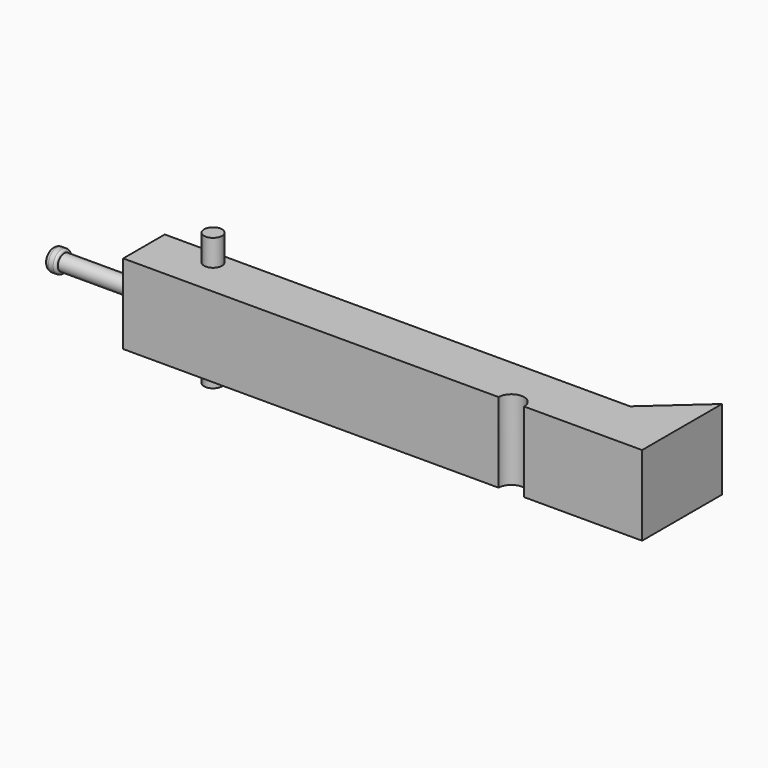
from build123d import *

# Parameters (mm, degrees)
F0_W          = 165.1
F0_H          = 25.4
F1_DEPTH      = 16.51
F3_R          = 2.8575
F4_DEPTH      = 8.382
F4_DEPTH_BACK = 33.782
F5_DEPTH      = 25.4
F6_DEPTH      = 25.4
F7_R          = 4.064
F8_DEPTH      = 25.4
F9_R          = 2.54
F10_DEPTH     = 25.4
F11_R         = 3.429
F12_DEPTH     = 3.81
F13_R         = 1.524
F14_R         = 0.762


# Not quite as in the source:
# - a feature names something its author has since deleted; it is built from what else it names


with BuildPart() as f1:
    # F0 (on Front) → F1 (new body)
    with BuildSketch(Plane.XZ):
        with Locations((17.2861106694, 1.5442719363)):
            Rectangle(F0_W, F0_H)
    extrude(amount=F1_DEPTH)

    # F3 (on face) → F4 (join, two sides)
    with BuildSketch(Plane(origin=(0, 0, -11.1557280637), x_dir=(1, 0, 0), z_dir=(0, 0, -1))) as f4_sk:
        with Locations((-46.4608334005, 4.2803706601)):
            Circle(F3_R)
    extrude(amount=F4_DEPTH)
    extrude(f4_sk.sketch, amount=-F4_DEPTH_BACK)

    # F2 (on face) → F5 (join)
    with BuildSketch(Plane(origin=(0, 0, -11.1557280637), x_dir=(1, 0, 0), z_dir=(0, 0, -1))):
        Polygon((99.8361106694, 0), (82.7972726808, 0), (99.8361106694, -15.24), align=None)
    extrude(amount=-F5_DEPTH)

    # F2 (on face) → F6 (join)
    with BuildSketch(Plane(origin=(0, 0, -11.1557280637), x_dir=(1, 0, 0), z_dir=(0, 0, -1))):
        Polygon((99.8361106694, 0), (82.7972726808, 0), (99.8361106694, -15.24), align=None)
    extrude(amount=-F6_DEPTH)

    # F7 (on face) → F8 (cut)
    with BuildSketch(Plane(origin=(0, 0, -11.1557280637), x_dir=(1, 0, 0), z_dir=(0, 0, -1))):
        with Locations((58.2425315266, 16.51)):
            Circle(F7_R)
    extrude(amount=-F8_DEPTH, mode=Mode.SUBTRACT)

    # F9 (on face) → F10 (join)
    with BuildSketch(Plane(origin=(-65.2638893306, 0, 0), x_dir=(0, -1, 0), z_dir=(-1, 0, 0))):
        with Locations((8.255, 1.5442719363)):
            Circle(F9_R)
    extrude(amount=F10_DEPTH)

    # F11 (on face) → F12 (join)
    with BuildSketch(Plane(origin=(-90.6638893306, 0, 0), x_dir=(0, -1, 0), z_dir=(-1, 0, 0))):
        with Locations((8.255, 1.5442719363)):
            Circle(F11_R)
    extrude(amount=F12_DEPTH)

    # F13
    f13_edges = [f1.edges().sort_by_distance(p)[0] for p in [
        (-94.473889, -4.826, 1.544272),
    ]]
    fillet(f13_edges, radius=F13_R)

    # F14
    f14_edges = [f1.edges().sort_by_distance(p)[0] for p in [
        (-90.663889, -4.826, 1.544272),
    ]]
    fillet(f14_edges, radius=F14_R)


solid = f1.part
